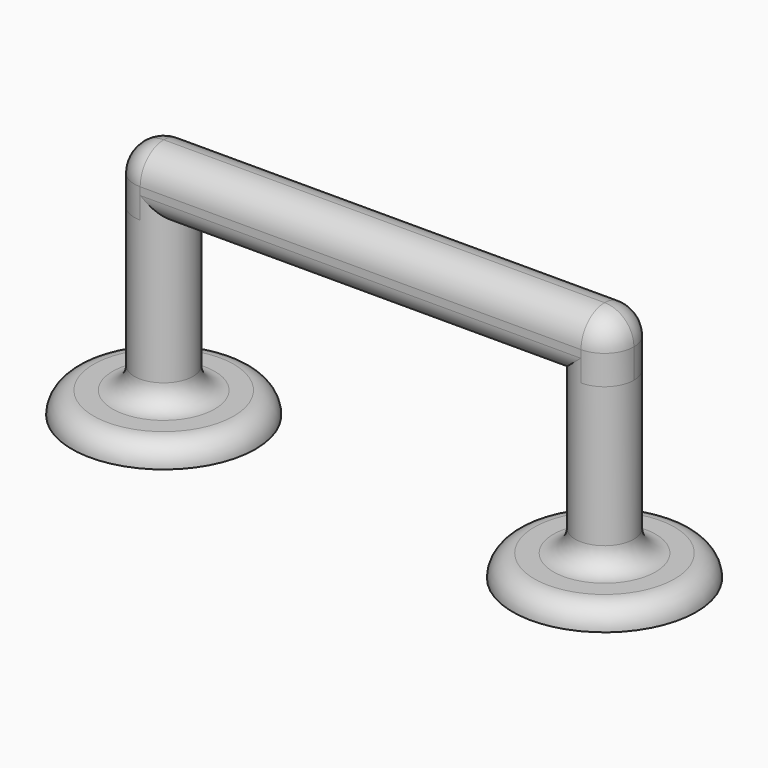
from build123d import *

# Parameters (mm, degrees)
F0_R         = 12.5
F1_DEPTH     = 3
F2_R         = 4
F3_DEPTH     = 30
F4_W         = 68
F4_H         = 8
F5_DEPTH     = 8
F6_R         = 3.9999
F7_T8_DEPTH  = 60
F7_S9_R      = 4
F7_T10_DEPTH = 32
F7_S11_R     = 4
F7_T12_DEPTH = 32
F7_T16_DEPTH = 60
F7_S17_R     = 4
F7_T18_DEPTH = 32
F7_S19_R     = 4
F7_T20_DEPTH = 32


# Not quite as in the source:
# - a fillet or chamfer that OpenCascade refuses, or shapes differently, is made with other operations: its cross-section is extruded or revolved along the edge and cut away or added
# - two fillets or chamfers of one size are made in one step
# - a fillet or chamfer is up to 0.001 mm smaller than in the source, because OpenCascade refuses the exact size


with BuildPart() as f1:
    # F0 (on Top) → F1 (new body)
    with BuildSketch(Plane.XY):
        with Locations((-30, 0)):
            Circle(F0_R)
    extrude(amount=F1_DEPTH)

    # F2 (on face) → F3 (join)
    with BuildSketch(Plane.XY.offset(3)):
        with Locations((-30, 0)):
            Circle(F2_R)
    extrude(amount=F3_DEPTH)



with BuildPart() as f1b:
    # F0 (on Top) → F1, piece 2 (new body)
    with BuildSketch(Plane.XY):
        with Locations((30, 0)):
            Circle(F0_R)
    extrude(amount=F1_DEPTH)

    # F2 (on face) → F3, piece 2 (join)
    with BuildSketch(Plane.XY.offset(3)):
        with Locations((30, 0)):
            Circle(F2_R)
    extrude(amount=F3_DEPTH)


with BuildPart() as f1_1:
    add(f1.part)

    add(f1b.part)  # F5 merges F1b
    # F4 (on face) → F5 (join)
    with BuildSketch(Plane.XY.offset(33)):
        Rectangle(F4_W, F4_H)
    extrude(amount=-F5_DEPTH)

    # F6 (radius 4 in the source; OpenCascade refuses exactly that, so slightly less here)
    f6_edges = [f1_1.edges().sort_by_distance(p)[0] for p in [
        (34, 0, 33),
        (0, 4, 33),
        (-34, 0, 33),
        (0, -4, 33),
        (34, -4, 29),
        (34, 4, 29),
        (-34, -4, 29),
        (-34, 4, 29),
    ]]
    fillet(f6_edges, radius=F6_R)

    # F7: fillet of radius 3 on 6 edges, made by hand

    # F7_s1 → F7_t2 (revolve)
    with BuildSketch(Plane.XZ):
        with BuildLine():
            ThreePointArc((33.9996, 6.0009656854), (34.8786796564, 3.8786796564), (37.0009656854, 2.9996))
            Line((37.0009656854, 2.9996), (37.0009656854, 2.6994634315))
            ThreePointArc((37.0009656854, 2.6994634315), (35.5004828427, 2.6998634315), (34, 2.6998634315))
            Line((34, 2.6998634315), (33.6998634315, 3))
            ThreePointArc((33.6998634315, 3), (33.6998634315, 4.5004828427), (33.6994634315, 6.0009656854))
            Line((33.6994634315, 6.0009656854), (33.9996, 6.0009656854))
        make_face()
    revolve(axis=Axis((30, 0, 3), (0, 0, 1)))

    # F7_s3 → F7_t4 (revolve)
    with BuildSketch(Plane.XZ):
        with BuildLine():
            ThreePointArc((-26.0004, 6.0009656854), (-25.1213203436, 3.8786796564), (-22.9990343146, 2.9996))
            Line((-22.9990343146, 2.9996), (-22.9990343146, 2.6994634315))
            ThreePointArc((-22.9990343146, 2.6994634315), (-24.4995171573, 2.6998634315), (-26, 2.6998634315))
            Line((-26, 2.6998634315), (-26.3001365685, 3))
            ThreePointArc((-26.3001365685, 3), (-26.3001365685, 4.5004828427), (-26.3005365685, 6.0009656854))
            Line((-26.3005365685, 6.0009656854), (-26.0004, 6.0009656854))
        make_face()
    revolve(axis=Axis((-30, 0, 3), (0, 0, 1)))


with BuildPart() as f7_tool6:
    # F7_s7 → F7_t8 (new body)
    with BuildSketch(Plane.YZ.offset(-30)):
        with BuildLine():
            ThreePointArc((-0.9990343146, 24.9996), (-3.1213203436, 25.8786796564), (-4.0004, 28.0009656854))
            Line((-4.0004, 28.0009656854), (-4.3005365685, 28.0009656854))
            ThreePointArc((-4.3005365685, 28.0009656854), (-4.3001365685, 26.5004828427), (-4.3001365685, 25))
            Line((-4.3001365685, 25), (-4, 24.6998634315))
            ThreePointArc((-4, 24.6998634315), (-2.4995171573, 24.6998634315), (-0.9990343146, 24.6994634315))
            Line((-0.9990343146, 24.6994634315), (-0.9990343146, 24.9996))
        make_face()
    extrude(amount=F7_T8_DEPTH)

    # F7_s9 → F7_t10 (cut, symmetric)
    with BuildSketch(Plane.XY.offset(26.4)):
        with Locations((30, 0)):
            Circle(F7_S9_R)
    extrude(amount=F7_T10_DEPTH, both=True, mode=Mode.SUBTRACT)

    # F7_s11 → F7_t12 (cut, symmetric)
    with BuildSketch(Plane.XY.offset(26.4)):
        with Locations((-30, 0)):
            Circle(F7_S11_R)
    extrude(amount=F7_T12_DEPTH, both=True, mode=Mode.SUBTRACT)


with BuildPart() as f1_2:
    add(f1_1.part)

    # F7_t5: cut F7_tool6
    add(f7_tool6.part, mode=Mode.SUBTRACT)


with BuildPart() as f7_tool14:
    # F7_s15 → F7_t16 (new body)
    with BuildSketch(Plane.YZ.offset(30)):
        with BuildLine():
            ThreePointArc((4.0004, 28.0009656854), (3.1213203436, 25.8786796564), (0.9990343146, 24.9996))
            Line((0.9990343146, 24.9996), (0.9990343146, 24.6994634315))
            ThreePointArc((0.9990343146, 24.6994634315), (2.4995171573, 24.6998634315), (4, 24.6998634315))
            Line((4, 24.6998634315), (4.3001365685, 25))
            ThreePointArc((4.3001365685, 25), (4.3001365685, 26.5004828427), (4.3005365685, 28.0009656854))
            Line((4.3005365685, 28.0009656854), (4.0004, 28.0009656854))
        make_face()
    extrude(amount=-F7_T16_DEPTH)

    # F7_s17 → F7_t18 (cut, symmetric)
    with BuildSketch(Plane.XY.offset(26.4)):
        with Locations((30, 0)):
            Circle(F7_S17_R)
    extrude(amount=F7_T18_DEPTH, both=True, mode=Mode.SUBTRACT)

    # F7_s19 → F7_t20 (cut, symmetric)
    with BuildSketch(Plane.XY.offset(26.4)):
        with Locations((-30, 0)):
            Circle(F7_S19_R)
    extrude(amount=F7_T20_DEPTH, both=True, mode=Mode.SUBTRACT)


with BuildPart() as f1_3:
    add(f1_2.part)

    # F7_t13: cut F7_tool14
    add(f7_tool14.part, mode=Mode.SUBTRACT)

    # F7_s21 → F7_t22 (revolve, cut)
    with BuildSketch(Plane.XZ):
        with BuildLine():
            ThreePointArc((39.4990343146, 3.0004), (41.6213203436, 2.1213203436), (42.5004, -0.0009656854))
            Line((42.5004, -0.0009656854), (42.8005365685, -0.0009656854))
            ThreePointArc((42.8005365685, -0.0009656854), (42.8001365685, 1.4995171573), (42.8001365685, 3))
            Line((42.8001365685, 3), (42.5, 3.3001365685))
            ThreePointArc((42.5, 3.3001365685), (40.9995171573, 3.3001365685), (39.4990343146, 3.3005365685))
            Line((39.4990343146, 3.3005365685), (39.4990343146, 3.0004))
        make_face()
    revolve(axis=Axis((30, 0, 3), (0, 0, 1)), mode=Mode.SUBTRACT)

    # F7_s23 → F7_t24 (revolve, cut)
    with BuildSketch(Plane.XZ):
        with BuildLine():
            ThreePointArc((-20.5009656854, 3.0004), (-18.3786796564, 2.1213203436), (-17.4996, -0.0009656854))
            Line((-17.4996, -0.0009656854), (-17.1994634315, -0.0009656854))
            ThreePointArc((-17.1994634315, -0.0009656854), (-17.1998634315, 1.4995171573), (-17.1998634315, 3))
            Line((-17.1998634315, 3), (-17.5, 3.3001365685))
            ThreePointArc((-17.5, 3.3001365685), (-19.0004828427, 3.3001365685), (-20.5009656854, 3.3005365685))
            Line((-20.5009656854, 3.3005365685), (-20.5009656854, 3.0004))
        make_face()
    revolve(axis=Axis((-30, 0, 3), (0, 0, 1)), mode=Mode.SUBTRACT)


solid = f1_3.part
